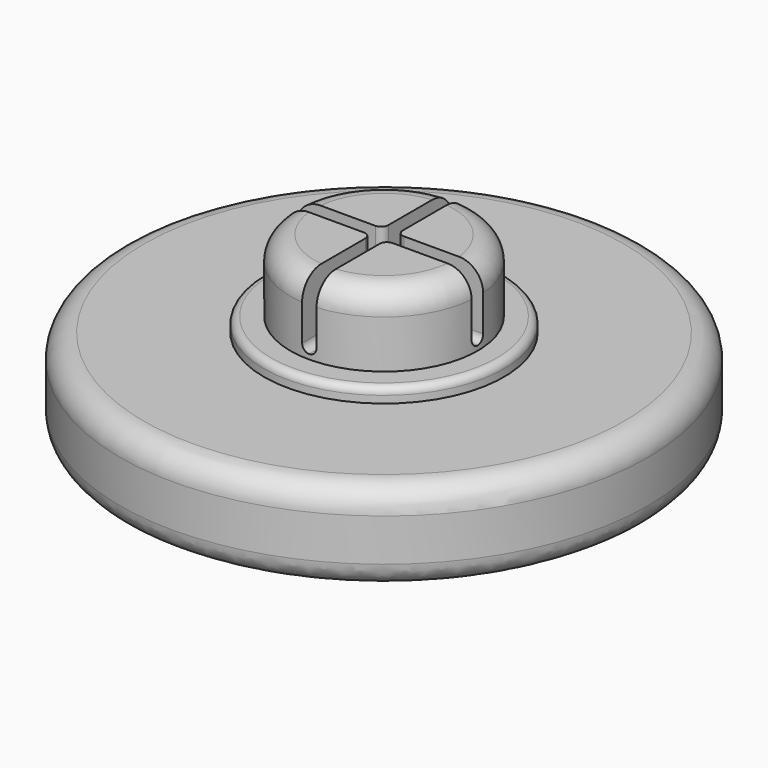
from build123d import *

# Parameters (mm, degrees)
F0_W     = 3.9
F0_H     = 3
F3_DEPTH = 2.8
F4_R     = 1
F5_R     = 0.2999


# Not quite as in the source:
# - a fillet or chamfer is up to 0.001 mm smaller than in the source, because OpenCascade refuses the exact size
# - a feature names something its author has since deleted; it is built from what else it names


with BuildPart() as f1:
    # F0 (on Front) → F1 (revolve)
    with BuildSketch(Plane.XZ):
        with Locations((-1.95, 6.1)):
            Rectangle(F0_W, F0_H)
        with BuildLine():
            Line((-11, 4), (-11, 0))
            ThreePointArc((-11, 0), (-5.533298022, 0.9052318686), (0, 1.2))
            Line((0, 1.2), (0, 4))
            Line((0, 4), (-5, 4))
            Line((-5, 4), (-11, 4))
        make_face()
        Polygon((-5, 4.6), (-5, 4), (0, 4), (0, 4.6), (-3.9, 4.6), align=None)
    revolve(axis=Axis((0, 0, 6.1), (0, 0, -1)))

    # F2 (on face) → F3 (cut)
    with BuildSketch(Plane.XY.offset(7.6)):
        with BuildLine():
            ThreePointArc((0.3, 3.888444419), (0, 3.9), (-0.3, 3.888444419))
            Line((-0.3, 3.888444419), (-0.3, 0.3))
            Line((-0.3, 0.3), (-3.888444419, 0.3))
            ThreePointArc((-3.888444419, 0.3), (-3.9, 0), (-3.888444419, -0.3))
            Line((-3.888444419, -0.3), (-0.3, -0.3))
            Line((-0.3, -0.3), (-0.3, -3.888444419))
            ThreePointArc((-0.3, -3.888444419), (0, -3.9), (0.3, -3.888444419))
            Line((0.3, -3.888444419), (0.3, -0.3))
            Line((0.3, -0.3), (3.888444419, -0.3))
            ThreePointArc((3.888444419, -0.3), (3.897110034, -0.150111235), (3.9, 0))
            ThreePointArc((3.9, 0), (3.897110034, 0.150111235), (3.888444419, 0.3))
            Line((3.888444419, 0.3), (0.3, 0.3))
            Line((0.3, 0.3), (0.3, 3.888444419))
        make_face()
    extrude(amount=-F3_DEPTH, mode=Mode.SUBTRACT)

    # F4
    f4_edges = [f1.edges().sort_by_distance(p)[0] for p in [
        (11, 0, 4),
        (11, 0, 0),
        (-2.757716, 2.757716, 7.6),
        (-2.757716, -2.757716, 7.6),
        (2.757716, -2.757716, 7.6),
        (2.757716, 2.757716, 7.6),
    ]]
    fillet(f4_edges, radius=F4_R)

    # F5 (radius 0.3 in the source; OpenCascade refuses exactly that, so slightly less here)
    f5_edges = [f1.edges().sort_by_distance(p)[0] for p in [
        (-2.094222, -0.3, 4.8),
        (2.094222, -0.3, 4.8),
        (2.094222, 0.3, 4.8),
        (-2.094222, 0.3, 4.8),
        (-0.3, -0.3, 6.2),
        (-0.3, 0.3, 6.2),
        (0.3, 0.3, 6.2),
        (0.3, -0.3, 6.2),
        (0.3, -2.094222, 4.8),
        (0.3, 2.094222, 4.8),
        (-0.3, 2.094222, 4.8),
        (-0.3, -2.094222, 4.8),
        (5, 0, 4.6),
    ]]
    fillet(f5_edges, radius=F5_R)


solid = f1.part
